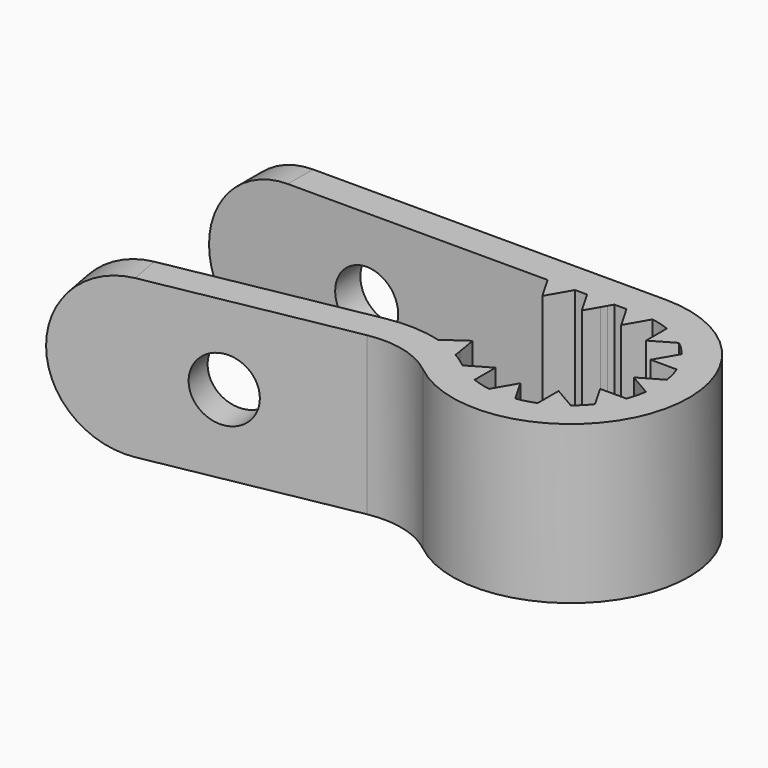
from build123d import *

# Parameters (mm, degrees)
F1_DEPTH = 10
F2_R     = 4.99999
F3_R     = 2
F4_DEPTH = 2
F5_R     = 2
F6_DEPTH = 2


# Not quite as in the source:
# - a fillet or chamfer is up to 0.001 mm smaller than in the source, because OpenCascade refuses the exact size


with BuildPart() as f1:
    # F0 (on Top) → F1 (new body)
    with BuildSketch(Plane.XY):
        Polygon((-5, 4), (-4.1339745962, 5.5), (-5.8660254038, 5.5), align=None)
        Polygon((-26.857039656, -8.0272581187), (-9.163588619, -4.7194203959), (-9.5311261437, -2.7534813918), (-27.2245771808, -6.0613191145), align=None)
        with BuildLine():
            ThreePointArc((-3.4370598373, -4.2937884991), (-2.75, -4.7631397208), (-2, -5.123475383))
            Line((-2, -5.123475383), (-2, -3.4641016151))
            Line((-2, -3.4641016151), (-3.4370598373, -4.2937884991))
        make_face()
        with BuildLine():
            ThreePointArc((-0.8296868839, -5.4370598373), (0, -5.5), (0.8296868839, -5.4370598373))
            Line((0.8296868839, -5.4370598373), (0, -4))
            Line((0, -4), (-0.8296868839, -5.4370598373))
        make_face()
        with BuildLine():
            ThreePointArc((2, -5.123475383), (2.75, -4.7631397208), (3.4370598373, -4.2937884991))
            Line((3.4370598373, -4.2937884991), (2, -3.4641016151))
            Line((2, -3.4641016151), (2, -5.123475383))
        make_face()
        with BuildLine():
            ThreePointArc((4.2937884991, -3.4370598373), (4.7631397208, -2.75), (5.123475383, -2))
            Line((5.123475383, -2), (3.4641016151, -2))
            Line((3.4641016151, -2), (4.2937884991, -3.4370598373))
        make_face()
        with BuildLine():
            ThreePointArc((5.4370598373, -0.8296868839), (5.5, 0), (5.4370598373, 0.8296868839))
            Line((5.4370598373, 0.8296868839), (4, 0))
            Line((4, 0), (5.4370598373, -0.8296868839))
        make_face()
        with BuildLine():
            Line((0, 4), (0.8296868839, 5.4370598373))
            ThreePointArc((0.8296868839, 5.4370598373), (0.416035392, 5.4842423864), (0, 5.5))
            Line((0, 5.5), (0, 4))
        make_face()
        with BuildLine():
            ThreePointArc((0, 5.5), (0.416035392, 5.4842423864), (0.8296868839, 5.4370598373))
            Line((0.8296868839, 5.4370598373), (0.8660254038, 5.5))
            Line((0.8660254038, 5.5), (0, 5.5))
        make_face()
        with BuildLine():
            Line((0, 4), (0, 5.5))
            ThreePointArc((0, 5.5), (-0.416035392, 5.4842423864), (-0.8296868839, 5.4370598373))
            Line((-0.8296868839, 5.4370598373), (0, 4))
        make_face()
        with BuildLine():
            Line((-2, 4.8660254038), (-1.8110659829, 5.1932687207))
            ThreePointArc((-1.8110659829, 5.1932687207), (-1.9058525019, 5.1592369824), (-2, 5.123475383))
            Line((-2, 5.123475383), (-2, 4.8660254038))
        make_face()
        with BuildLine():
            Line((-2, 4.8660254038), (-2, 5.123475383))
            ThreePointArc((-2, 5.123475383), (-2.4559554031, 4.9212074797), (-2.8917104606, 4.6784624196))
            Line((-2.8917104606, 4.6784624196), (-2.5, 4))
            Line((-2.5, 4), (-2, 4.8660254038))
        make_face()
        with BuildLine():
            ThreePointArc((-9.163588619, -4.7194203959), (-6.8106363862, -4.7920452574), (-4.7035733226, -5.8417803792))
            ThreePointArc((-4.7035733226, -5.8417803792), (-6.0524247462, -4.4292386131), (-6.9908223073, -2.7163216797))
            ThreePointArc((-6.9908223073, -2.7163216797), (-8.2625591256, -2.6265549538), (-9.5311261437, -2.7534813918))
            Line((-9.5311261437, -2.7534813918), (-9.163588619, -4.7194203959))
        make_face()
        with BuildLine():
            Line((-4.6842221141, -1.9200455203), (-4.9155419039, -2.4672753781))
            ThreePointArc((-4.9155419039, -2.4672753781), (-4.7096941165, -2.8405600379), (-4.4755547297, -3.196781172))
            Line((-4.4755547297, -3.196781172), (-4.6842221141, -1.9200455203))
        make_face()
        with BuildLine():
            Line((-4.6842221141, -1.9200455203), (-5.0512472947, -2.175982713))
            ThreePointArc((-5.0512472947, -2.175982713), (-4.9855224988, -2.3226203765), (-4.9155419039, -2.4672753781))
            Line((-4.9155419039, -2.4672753781), (-4.6842221141, -1.9200455203))
        make_face()
        with BuildLine():
            ThreePointArc((-0.8296868839, 5.4370598373), (-0.416035392, 5.4842423864), (0, 5.5))
            Line((0, 5.5), (-0.8660254038, 5.5))
            Line((-0.8660254038, 5.5), (-0.8296868839, 5.4370598373))
        make_face()
        with BuildLine():
            Line((-5.0512472947, -2.175982713), (-6.104954117, -2.9107627231))
            ThreePointArc((-6.104954117, -2.9107627231), (-5.6640980624, -3.0507217811), (-5.2327078262, -3.2175901813))
            Line((-5.2327078262, -3.2175901813), (-4.9155419039, -2.4672753781))
            ThreePointArc((-4.9155419039, -2.4672753781), (-4.9855224988, -2.3226203765), (-5.0512472947, -2.175982713))
        make_face()
        with BuildLine():
            ThreePointArc((-2, 5.123475383), (-1.9058525019, 5.1592369824), (-1.8110659829, 5.1932687207))
            Line((-1.8110659829, 5.1932687207), (-1.6339745962, 5.5))
            Line((-1.6339745962, 5.5), (-3.3660254038, 5.5))
            Line((-3.3660254038, 5.5), (-2.8917104606, 4.6784624196))
            ThreePointArc((-2.8917104606, 4.6784624196), (-2.4559554031, 4.9212074797), (-2, 5.123475383))
        make_face()
        with BuildLine():
            Line((-4.9155419039, -2.4672753781), (-5.2327078262, -3.2175901813))
            ThreePointArc((-5.2327078262, -3.2175901813), (-4.8124241684, -3.4107332523), (-4.404845606, -3.629416389))
            Line((-4.404845606, -3.629416389), (-4.4755547297, -3.196781172))
            ThreePointArc((-4.4755547297, -3.196781172), (-4.7096941165, -2.8405600379), (-4.9155419039, -2.4672753781))
        make_face()
        with BuildLine():
            ThreePointArc((0.8296868839, 5.4370598373), (1.4235047481, 5.3125920446), (2, 5.123475383))
            Line((2, 5.123475383), (2, 3.4641016151))
            Line((2, 3.4641016151), (3.4370598373, 4.2937884991))
            ThreePointArc((3.4370598373, 4.2937884991), (3.8890872965, 3.8890872965), (4.2937884991, 3.4370598373))
            Line((4.2937884991, 3.4370598373), (3.4641016151, 2))
            Line((3.4641016151, 2), (5.123475383, 2))
            ThreePointArc((5.123475383, 2), (5.3125920446, 1.4235047481), (5.4370598373, 0.8296868839))
            ThreePointArc((5.4370598373, 0.8296868839), (5.5, 0), (5.4370598373, -0.8296868839))
            ThreePointArc((5.4370598373, -0.8296868839), (5.3125920446, -1.4235047481), (5.123475383, -2))
            ThreePointArc((5.123475383, -2), (4.7631397208, -2.75), (4.2937884991, -3.4370598373))
            ThreePointArc((4.2937884991, -3.4370598373), (3.8890872965, -3.8890872965), (3.4370598373, -4.2937884991))
            ThreePointArc((3.4370598373, -4.2937884991), (2.75, -4.7631397208), (2, -5.123475383))
            ThreePointArc((2, -5.123475383), (1.4235047481, -5.3125920446), (0.8296868839, -5.4370598373))
            ThreePointArc((0.8296868839, -5.4370598373), (0, -5.5), (-0.8296868839, -5.4370598373))
            ThreePointArc((-0.8296868839, -5.4370598373), (-1.4235047481, -5.3125920446), (-2, -5.123475383))
            ThreePointArc((-2, -5.123475383), (-2.75, -4.7631397208), (-3.4370598373, -4.2937884991))
            ThreePointArc((-3.4370598373, -4.2937884991), (-3.4431769685, -4.2888847459), (-3.4492871033, -4.2839722781))
            ThreePointArc((-3.4492871033, -4.2839722781), (-3.9144118435, -3.9382205471), (-4.404845606, -3.629416389))
            ThreePointArc((-4.404845606, -3.629416389), (-4.8124241684, -3.4107332523), (-5.2327078262, -3.2175901813))
            ThreePointArc((-5.2327078262, -3.2175901813), (-5.6640980624, -3.0507217811), (-6.104954117, -2.9107627231))
            ThreePointArc((-6.104954117, -2.9107627231), (-6.544946362, -2.800139211), (-6.9908223073, -2.7163216797))
            ThreePointArc((-6.9908223073, -2.7163216797), (-6.0524247462, -4.4292386131), (-4.7035733226, -5.8417803792))
            ThreePointArc((-4.7035733226, -5.8417803792), (7.0733073185, -2.493656668), (0, 7.5))
            Line((0, 7.5), (-27.3435036541, 7.5))
            Line((-27.3435036541, 7.5), (-27.3435036541, 5.5))
            Line((-27.3435036541, 5.5), (-5.8660254038, 5.5))
            Line((-5.8660254038, 5.5), (-4.1339745962, 5.5))
            Line((-4.1339745962, 5.5), (-3.3660254038, 5.5))
            Line((-3.3660254038, 5.5), (-1.6339745962, 5.5))
            Line((-1.6339745962, 5.5), (-0.8660254038, 5.5))
            Line((-0.8660254038, 5.5), (0, 5.5))
            Line((0, 5.5), (0.8660254038, 5.5))
            Line((0.8660254038, 5.5), (0.8296868839, 5.4370598373))
        make_face()
    extrude(amount=F1_DEPTH)

    # F2 (radius 5 in the source; OpenCascade refuses exactly that, so slightly less here)
    f2_edges = [f1.edges().sort_by_distance(p)[0] for p in [
        (-27.343504, 6.5, 10),
        (-27.343504, 6.5, 0),
        (-27.040808, -7.044289, 0),
        (-27.040808, -7.044289, 10),
    ]]
    fillet(f2_edges, radius=F2_R)

    # F3 (on face) → F4 (cut)
    with BuildSketch(Plane(origin=(0.5430486336, -2.9047387492, 0), x_dir=(0.9829695021, 0.1837687624, 0), z_dir=(0.1837687624, -0.9829695021, 0))):
        with Locations((-17.8748101871, 5)):
            Circle(F3_R)
    extrude(amount=-F4_DEPTH, mode=Mode.SUBTRACT)

    # F5 (on face) → F6 (cut)
    with BuildSketch(Plane(origin=(0, 7.5, 0), x_dir=(-1, 0, 0), z_dir=(0, 1, 0))):
        with Locations((17.3435036541, 5)):
            Circle(F5_R)
    extrude(amount=-F6_DEPTH, mode=Mode.SUBTRACT)


solid = f1.part
